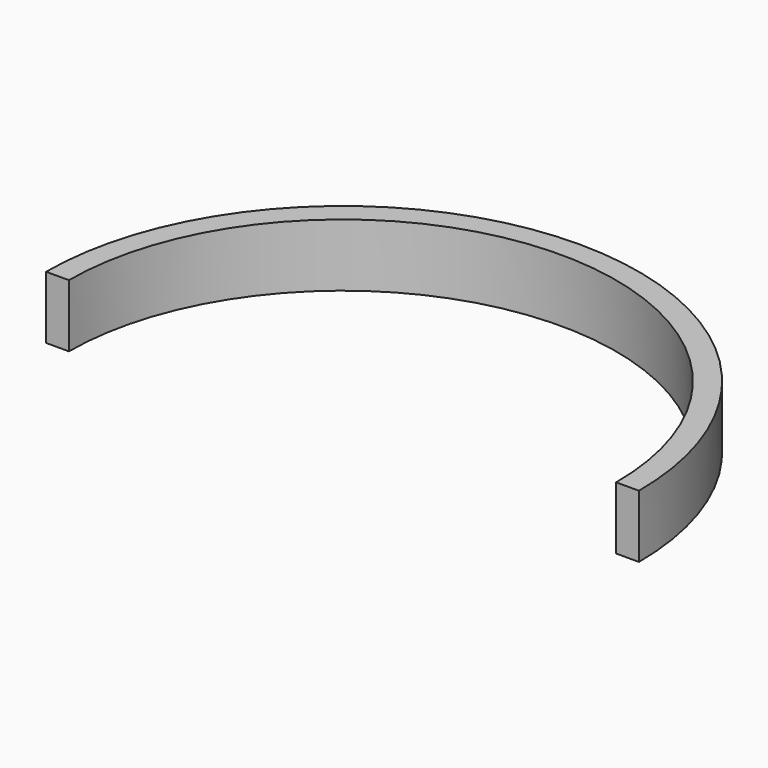
from build123d import *

# Parameters (mm, degrees)
F1_DEPTH = 5.5


with BuildPart() as f1:
    # F0 (on Top) → F1 (new body)
    with BuildSketch(Plane.XY):
        with BuildLine():
            Line((24, 0), (26, 0))
            ThreePointArc((26, 0), (0, 26), (-26, 0))
            Line((-26, 0), (-24, 0))
            ThreePointArc((-24, 0), (0, 24), (24, 0))
        make_face()
    extrude(amount=F1_DEPTH)


solid = f1.part
